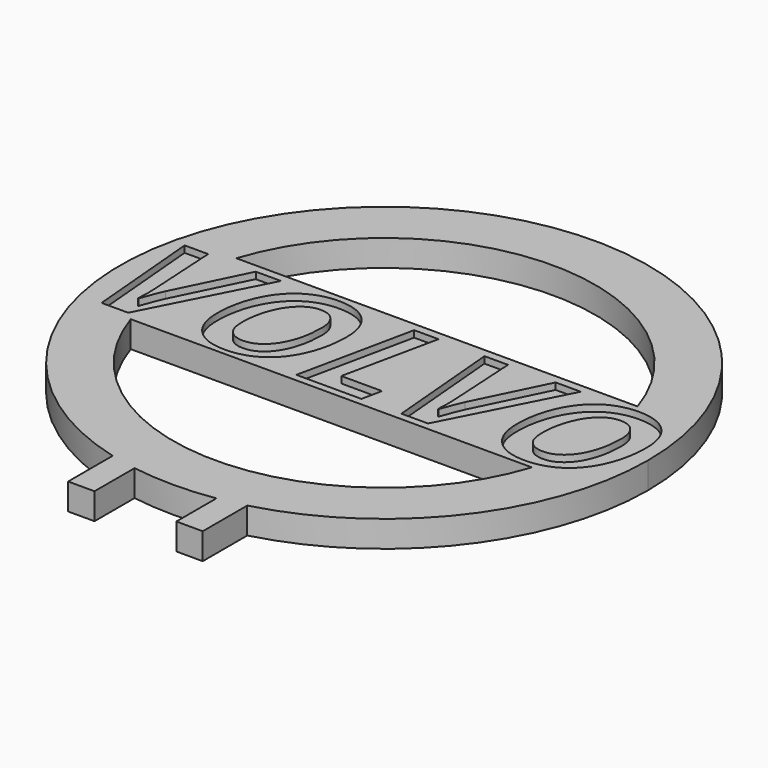
from build123d import *

# Parameters (mm, degrees)
F1_DEPTH     = 2
F2_TEXT_SIZE = 12.3611111111
F3_DEPTH     = 0.5


# Not quite as in the source:
# - Text() gives the source's letters only with a copy of the font that has no kerning and outlines rounded to 1/6400 em; it was checked with that copy


with BuildPart() as f1:
    # F0 (on Top) → F1 (new body)
    with BuildSketch(Plane.XY):
        with BuildLine():
            ThreePointArc((5.1, -19.3388210602), (15.8429795178, -12.2065556157), (20, 0))
            ThreePointArc((20, 0), (-12.2065556157, 15.8429795178), (-5.1, -19.3388210602))
            ThreePointArc((-5.1, -19.3388210602), (-4.1053609369, -19.5741158569), (-3.1, -19.7582893996))
            ThreePointArc((-3.1, -19.7582893996), (0, -20), (3.1, -19.7582893996))
            ThreePointArc((3.1, -19.7582893996), (4.1053609369, -19.5741158569), (5.1, -19.3388210602))
        make_face()
        with BuildLine():
            ThreePointArc((15.1986841536, 5), (15.7984009706, 2.5319018092), (16, 0))
            ThreePointArc((16, 0), (15.7984009706, -2.5319018092), (15.1986841536, -5))
            ThreePointArc((15.1986841536, -5), (0, -16), (-15.1986841536, -5))
            ThreePointArc((-15.1986841536, -5), (-15.7984009706, -2.5319018092), (-16, 0))
            ThreePointArc((-16, 0), (-15.7984009706, 2.5319018092), (-15.1986841536, 5))
            ThreePointArc((-15.1986841536, 5), (0, 16), (15.1986841536, 5))
        make_face(mode=Mode.SUBTRACT)
        with BuildLine():
            ThreePointArc((-3.1, -19.7582893996), (-4.1053609369, -19.5741158569), (-5.1, -19.3388210602))
            Line((-5.1, -19.3388210602), (-5.1, -23.5549743987))
            Line((-5.1, -23.5549743987), (-3.1, -23.5549743987))
            Line((-3.1, -23.5549743987), (-3.1, -19.7582893996))
        make_face()
        with BuildLine():
            Line((5.1, -23.5549743987), (5.1, -19.3388210602))
            ThreePointArc((5.1, -19.3388210602), (4.1053609369, -19.5741158569), (3.1, -19.7582893996))
            Line((3.1, -19.7582893996), (3.1, -23.5549743987))
            Line((3.1, -23.5549743987), (5.1, -23.5549743987))
        make_face()
        with BuildLine():
            Line((0, 0), (16, 0))
            ThreePointArc((16, 0), (15.7984009706, 2.5319018092), (15.1986841536, 5))
            Line((15.1986841536, 5), (0, 5))
            Line((0, 5), (-15.1986841536, 5))
            ThreePointArc((-15.1986841536, 5), (-15.7984009706, 2.5319018092), (-16, 0))
            Line((-16, 0), (0, 0))
        make_face()
        with BuildLine():
            ThreePointArc((15.1986841536, -5), (15.7984009706, -2.5319018092), (16, 0))
            Line((16, 0), (0, 0))
            Line((0, 0), (-16, 0))
            ThreePointArc((-16, 0), (-15.7984009706, -2.5319018092), (-15.1986841536, -5))
            Line((-15.1986841536, -5), (0, -5))
            Line((0, -5), (15.1986841536, -5))
        make_face()
    extrude(amount=F1_DEPTH)

    # F2 (on face) → F3 (cut)
    with BuildSketch(Plane.XY.offset(2)):
        with Locations((-19.7275607639, -4.4480884294)):
            Text('VOLVO', F2_TEXT_SIZE, font='Open Sans', font_style=FontStyle.BOLDITALIC, text_align=(TextAlign.LEFT, TextAlign.BOTTOM))
    extrude(amount=-F3_DEPTH, mode=Mode.SUBTRACT)


solid = f1.part
